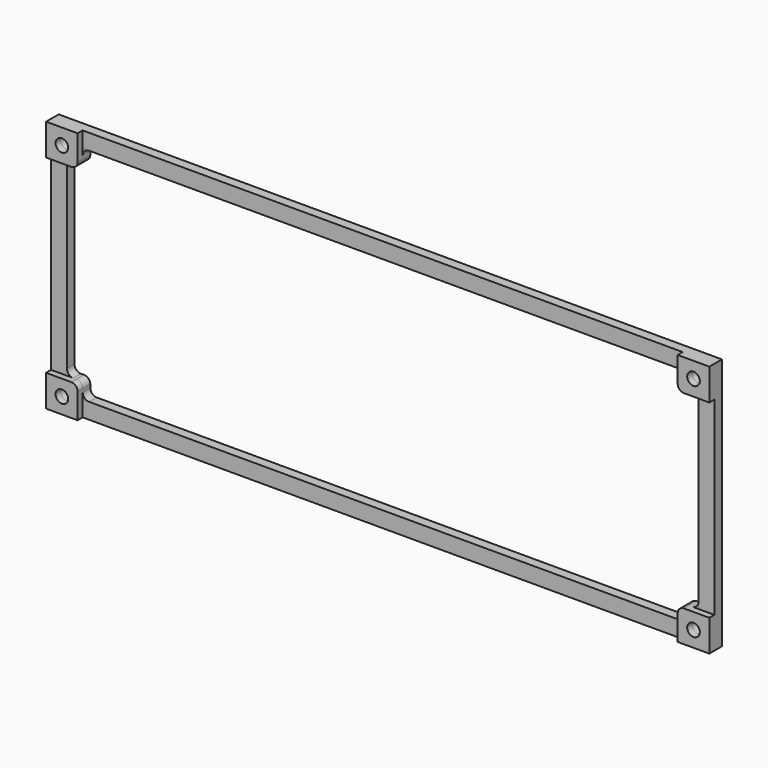
from build123d import *

# Parameters (mm, degrees)
F0_W        = 210
F0_H        = 80
F1_DEPTH    = 3
F2_R        = 2
F3_DEPTH    = 25
F4_W        = 10
F4_H        = 10
F4_R        = 2
F5_DEPTH    = 2
F6_W        = 5
F6_H        = 60
F7_DEPTH    = 25
F8_T1_DEPTH = 3
F8_T3_DEPTH = 7
F8_T5_DEPTH = 8
F8_T7_DEPTH = 15


# Not quite as in the source:
# - a fillet or chamfer that OpenCascade refuses, or shapes differently, is made with other operations: its cross-section is extruded or revolved along the edge and cut away or added


with BuildPart() as f1:
    # F0 (on Front) → F1 (new body)
    with BuildSketch(Plane.XZ):
        Rectangle(F0_W, F0_H)
    extrude(amount=F1_DEPTH)

    # F2 (on face) → F3 (cut)
    with BuildSketch(Plane.XZ.offset(3)):
        with Locations((-100.000000149, 35.000000149)):
            Circle(F2_R)
        with Locations((-100.000000149, -35.000000149)):
            Circle(F2_R)
        with Locations((100.000000149, -35.000000149)):
            Circle(F2_R)
        with Locations((100.000000149, 35.000000149)):
            Circle(F2_R)
    extrude(amount=-F3_DEPTH, mode=Mode.SUBTRACT)

    # F4 (on face) → F5 (join)
    with BuildSketch(Plane.XZ.offset(3)):
        with Locations((-100, 35)):
            Rectangle(F4_W, F4_H)
        with Locations((-100.000000149, 35.000000149)):
            Circle(F4_R, mode=Mode.SUBTRACT)
        with Locations((-100, -35)):
            Rectangle(F4_W, F4_H)
        with Locations((-100.000000149, -35.000000149)):
            Circle(F4_R, mode=Mode.SUBTRACT)
        with Locations((100, -35)):
            Rectangle(F4_W, F4_H)
        with Locations((100.000000149, -35.000000149)):
            Circle(F4_R, mode=Mode.SUBTRACT)
        with Locations((100, 35)):
            Rectangle(F4_W, F4_H)
        with Locations((100.000000149, 35.000000149)):
            Circle(F4_R, mode=Mode.SUBTRACT)
    extrude(amount=F5_DEPTH)

    # F6 (on face) → F7 (cut)
    with BuildSketch(Plane.XZ.offset(3)):
        Polygon((95, 35), (-95, 35), (-95, 30), (-95, -30), (-95, -35), (95, -35), (95, -30), (95, 30), align=None)
        with Locations((-97.5, 0)):
            Rectangle(F6_W, F6_H)
        with Locations((97.5, 0)):
            Rectangle(F6_W, F6_H)
    extrude(amount=-F7_DEPTH, mode=Mode.SUBTRACT)

    # F8: fillet of radius 2 on 15 edges, made by hand

    # F8_s2 → F8_t1 (join)
    with BuildSketch(Plane.XZ):
        with BuildLine():
            ThreePointArc((-100, 28), (-99.4142135624, 29.4142135624), (-98, 30))
            Line((-98, 30), (-100, 30))
            Line((-100, 30), (-100, 28))
        make_face()
        with BuildLine():
            ThreePointArc((-95, 33), (-94.4142135624, 34.4142135624), (-93, 35))
            Line((-93, 35), (-95, 35))
            Line((-95, 35), (-95, 33))
        make_face()
        with BuildLine():
            ThreePointArc((-98, -30), (-99.4142135624, -29.4142135624), (-100, -28))
            Line((-100, -28), (-100, -30))
            Line((-100, -30), (-98, -30))
        make_face()
        with BuildLine():
            ThreePointArc((-93, -35), (-94.4142135624, -34.4142135624), (-95, -33))
            Line((-95, -33), (-95, -35))
            Line((-95, -35), (-93, -35))
        make_face()
        with BuildLine():
            ThreePointArc((95, 33), (94.4142135624, 34.4142135624), (93, 35))
            Line((93, 35), (95, 35))
            Line((95, 35), (95, 33))
        make_face()
        with BuildLine():
            ThreePointArc((100, 28), (99.4142135624, 29.4142135624), (98, 30))
            Line((98, 30), (100, 30))
            Line((100, 30), (100, 28))
        make_face()
        with BuildLine():
            ThreePointArc((95, -33), (94.4142135624, -34.4142135624), (93, -35))
            Line((93, -35), (95, -35))
            Line((95, -35), (95, -33))
        make_face()
        with BuildLine():
            ThreePointArc((100, -28), (99.4142135624, -29.4142135624), (98, -30))
            Line((98, -30), (100, -30))
            Line((100, -30), (100, -28))
        make_face()
    extrude(amount=F8_T1_DEPTH)

    # F8_s4 → F8_t3 (cut)
    with BuildSketch(Plane.XZ.offset(3)):
        with BuildLine():
            ThreePointArc((-95, 32), (-95.5857864376, 30.5857864376), (-97, 30))
            Line((-97, 30), (-95, 30))
            Line((-95, 30), (-95, 32))
        make_face()
        with BuildLine():
            ThreePointArc((-97, -30), (-95.5857864376, -30.5857864376), (-95, -32))
            Line((-95, -32), (-95, -30))
            Line((-95, -30), (-97, -30))
        make_face()
        with BuildLine():
            ThreePointArc((95, 32), (95.5857864376, 30.5857864376), (97, 30))
            Line((97, 30), (95, 30))
            Line((95, 30), (95, 32))
        make_face()
    extrude(amount=F8_T3_DEPTH, mode=Mode.SUBTRACT)

    # F8_s6 → F8_t5 (cut)
    with BuildSketch(Plane.XZ.offset(-5)):
        with BuildLine():
            ThreePointArc((-95, 32), (-95.5857864376, 30.5857864376), (-97, 30))
            Line((-97, 30), (-95, 30))
            Line((-95, 30), (-95, 32))
        make_face()
        with BuildLine():
            ThreePointArc((-97, -30), (-95.5857864376, -30.5857864376), (-95, -32))
            Line((-95, -32), (-95, -30))
            Line((-95, -30), (-97, -30))
        make_face()
        with BuildLine():
            ThreePointArc((95, 32), (95.5857864376, 30.5857864376), (97, 30))
            Line((97, 30), (95, 30))
            Line((95, 30), (95, 32))
        make_face()
    extrude(amount=F8_T5_DEPTH, mode=Mode.SUBTRACT)

    # F8_s8 → F8_t7 (cut)
    with BuildSketch(Plane.XZ.offset(-5)):
        with BuildLine():
            ThreePointArc((95, -32), (95.5857864376, -30.5857864376), (97, -30))
            Line((97, -30), (95, -30))
            Line((95, -30), (95, -32))
        make_face()
    extrude(amount=F8_T7_DEPTH, mode=Mode.SUBTRACT)


solid = f1.part
